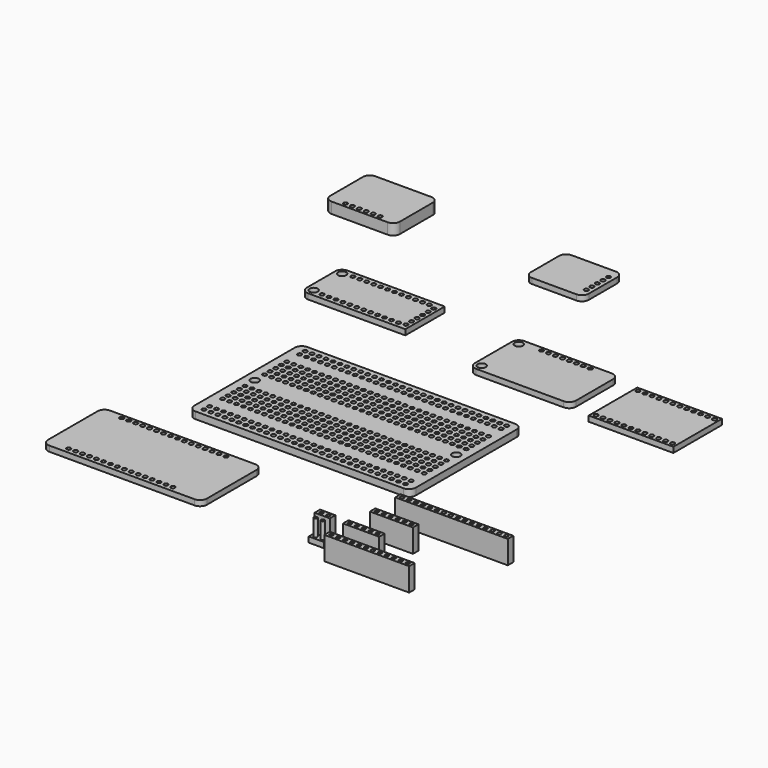
from build123d import *

# Parameters (mm, degrees)
F0_W      = 81
F0_H      = 51
F0_R      = 0.75
F0_R_2    = 1.5
F1_DEPTH  = 2.5
F2_R      = 2.5
F3_W      = 5.58
F3_H      = 2.5
F3_R      = 0.625
F4_DEPTH  = 8.5
F5_DEPTH  = 2
F6_W      = 37
F6_H      = 22
F6_R      = 1.5
F6_R_2    = 0.75
F7_DEPTH  = 2
F8_R      = 2.5
F3_W_2    = 13.2
F9_DEPTH  = 8.5
F6_W_2    = 38
F6_H_2    = 18
F10_DEPTH = 2
F11_R     = 2.5
F3_W_3    = 30.98
F12_DEPTH = 8.5
F6_W_3    = 58.08
F6_H_3    = 27.72
F13_DEPTH = 2
F14_R     = 2.54
F6_W_4    = 21.2070047855
F15_DEPTH = 2
F16_R     = 2.5
F6_W_5    = 25.5
F6_H_4    = 20
F17_DEPTH = 4
F18_R     = 2.5
F6_W_6    = 30.9399995804
F6_H_5    = 22.16
F19_DEPTH = 2
F3_W_4    = 15.74
F20_DEPTH = 8.5
F21_DEPTH = 8
F3_W_5    = 41.14
F3_R_2    = 0.6724855027
F22_DEPTH = 8.5


# Not quite as in the source:
# - a feature names something its author has since deleted; it is built from what else it names


with BuildPart() as f1:
    # F0 (on Top) → F1 (new body)
    with BuildSketch(Plane.XY):
        with Locations((2.4331173706, -0.0898422903)):
            Rectangle(F0_W, F0_H)
        with Locations((-34.3968826294, -23.1898422903)):
            Circle(F0_R, mode=Mode.SUBTRACT)
        with Locations((-31.8568826675, -23.1898422903)):
            Circle(F0_R, mode=Mode.SUBTRACT)
        with Locations((-29.3168827057, -23.1898422903)):
            Circle(F0_R, mode=Mode.SUBTRACT)
        with Locations((-34.3968826772, -20.6498423284)):
            Circle(F0_R, mode=Mode.SUBTRACT)
        with Locations((-31.8568827154, -20.6498423284)):
            Circle(F0_R, mode=Mode.SUBTRACT)
        with Locations((-29.3168827535, -20.6498423284)):
            Circle(F0_R, mode=Mode.SUBTRACT)
        with Locations((-26.7768827438, -23.1898422903)):
            Circle(F0_R, mode=Mode.SUBTRACT)
        with Locations((-24.236882782, -23.1898422903)):
            Circle(F0_R, mode=Mode.SUBTRACT)
        with Locations((-21.6968828201, -23.1898422903)):
            Circle(F0_R, mode=Mode.SUBTRACT)
        with Locations((-19.1568828583, -23.1898422903)):
            Circle(F0_R, mode=Mode.SUBTRACT)
        with Locations((-26.7768827917, -20.6498423284)):
            Circle(F0_R, mode=Mode.SUBTRACT)
        with Locations((-24.2368828298, -20.6498423284)):
            Circle(F0_R, mode=Mode.SUBTRACT)
        with Locations((-21.696882868, -20.6498423284)):
            Circle(F0_R, mode=Mode.SUBTRACT)
        with Locations((-19.1568829061, -20.6498423284)):
            Circle(F0_R, mode=Mode.SUBTRACT)
        with Locations((-34.3968826584, -14.6599998474)):
            Circle(F0_R, mode=Mode.SUBTRACT)
        with Locations((-31.8568826966, -14.6599998474)):
            Circle(F0_R, mode=Mode.SUBTRACT)
        with Locations((-29.3168827347, -14.6599998474)):
            Circle(F0_R, mode=Mode.SUBTRACT)
        with Locations((-26.7768827729, -14.6599998474)):
            Circle(F0_R, mode=Mode.SUBTRACT)
        with Locations((-24.236882811, -14.6599998474)):
            Circle(F0_R, mode=Mode.SUBTRACT)
        with Locations((-21.6968828492, -14.6599998474)):
            Circle(F0_R, mode=Mode.SUBTRACT)
        with Locations((-19.1568828873, -14.6599998474)):
            Circle(F0_R, mode=Mode.SUBTRACT)
        with Locations((-16.6168828964, -23.1898422903)):
            Circle(F0_R, mode=Mode.SUBTRACT)
        with Locations((-14.0768829346, -23.1898422903)):
            Circle(F0_R, mode=Mode.SUBTRACT)
        with Locations((-11.5368829727, -23.1898422903)):
            Circle(F0_R, mode=Mode.SUBTRACT)
        with Locations((-8.9968830109, -23.1898422903)):
            Circle(F0_R, mode=Mode.SUBTRACT)
        with Locations((-16.6168829443, -20.6498423284)):
            Circle(F0_R, mode=Mode.SUBTRACT)
        with Locations((-14.0768829824, -20.6498423284)):
            Circle(F0_R, mode=Mode.SUBTRACT)
        with Locations((-11.5368830206, -20.6498423284)):
            Circle(F0_R, mode=Mode.SUBTRACT)
        with Locations((-8.9968830587, -20.6498423284)):
            Circle(F0_R, mode=Mode.SUBTRACT)
        with Locations((-6.456883049, -23.1898422903)):
            Circle(F0_R, mode=Mode.SUBTRACT)
        with Locations((-3.9168830872, -23.1898422903)):
            Circle(F0_R, mode=Mode.SUBTRACT)
        with Locations((-1.3768831253, -23.1898422903)):
            Circle(F0_R, mode=Mode.SUBTRACT)
        with Locations((1.1631168365, -23.1898422903)):
            Circle(F0_R, mode=Mode.SUBTRACT)
        with Locations((-6.4568830969, -20.6498423284)):
            Circle(F0_R, mode=Mode.SUBTRACT)
        with Locations((-3.916883135, -20.6498423284)):
            Circle(F0_R, mode=Mode.SUBTRACT)
        with Locations((-1.3768831731, -20.6498423284)):
            Circle(F0_R, mode=Mode.SUBTRACT)
        with Locations((1.1631167887, -20.6498423284)):
            Circle(F0_R, mode=Mode.SUBTRACT)
        with Locations((-16.6168829255, -14.6599998474)):
            Circle(F0_R, mode=Mode.SUBTRACT)
        with Locations((-14.0768829636, -14.6599998474)):
            Circle(F0_R, mode=Mode.SUBTRACT)
        with Locations((-11.5368830018, -14.6599998474)):
            Circle(F0_R, mode=Mode.SUBTRACT)
        with Locations((-8.9968830399, -14.6599998474)):
            Circle(F0_R, mode=Mode.SUBTRACT)
        with Locations((-6.4568830781, -14.6599998474)):
            Circle(F0_R, mode=Mode.SUBTRACT)
        with Locations((-3.9168831162, -14.6599998474)):
            Circle(F0_R, mode=Mode.SUBTRACT)
        with Locations((-1.3768831544, -14.6599998474)):
            Circle(F0_R, mode=Mode.SUBTRACT)
        with Locations((1.1631168075, -14.6599998474)):
            Circle(F0_R, mode=Mode.SUBTRACT)
        with Locations((-34.3968826584, -12.1199998856)):
            Circle(F0_R, mode=Mode.SUBTRACT)
        with Locations((-31.8568826966, -12.1199998856)):
            Circle(F0_R, mode=Mode.SUBTRACT)
        with Locations((-29.3168827347, -12.1199998856)):
            Circle(F0_R, mode=Mode.SUBTRACT)
        with Locations((-34.3968826584, -9.5799999237)):
            Circle(F0_R, mode=Mode.SUBTRACT)
        with Locations((-34.3968826584, -7.0399999619)):
            Circle(F0_R, mode=Mode.SUBTRACT)
        with Locations((-31.8568826966, -9.5799999237)):
            Circle(F0_R, mode=Mode.SUBTRACT)
        with Locations((-29.3168827347, -9.5799999237)):
            Circle(F0_R, mode=Mode.SUBTRACT)
        with Locations((-31.8568826966, -7.0399999619)):
            Circle(F0_R, mode=Mode.SUBTRACT)
        with Locations((-29.3168827347, -7.0399999619)):
            Circle(F0_R, mode=Mode.SUBTRACT)
        with Locations((-26.7768827729, -12.1199998856)):
            Circle(F0_R, mode=Mode.SUBTRACT)
        with Locations((-24.236882811, -12.1199998856)):
            Circle(F0_R, mode=Mode.SUBTRACT)
        with Locations((-21.6968828492, -12.1199998856)):
            Circle(F0_R, mode=Mode.SUBTRACT)
        with Locations((-19.1568828873, -12.1199998856)):
            Circle(F0_R, mode=Mode.SUBTRACT)
        with Locations((-26.7768827729, -9.5799999237)):
            Circle(F0_R, mode=Mode.SUBTRACT)
        with Locations((-24.236882811, -9.5799999237)):
            Circle(F0_R, mode=Mode.SUBTRACT)
        with Locations((-26.7768827729, -7.0399999619)):
            Circle(F0_R, mode=Mode.SUBTRACT)
        with Locations((-24.236882811, -7.0399999619)):
            Circle(F0_R, mode=Mode.SUBTRACT)
        with Locations((-21.6968828492, -9.5799999237)):
            Circle(F0_R, mode=Mode.SUBTRACT)
        with Locations((-19.1568828873, -9.5799999237)):
            Circle(F0_R, mode=Mode.SUBTRACT)
        with Locations((-21.6968828492, -7.0399999619)):
            Circle(F0_R, mode=Mode.SUBTRACT)
        with Locations((-19.1568828873, -7.0399999619)):
            Circle(F0_R, mode=Mode.SUBTRACT)
        with Locations((-34.3968826584, -4.5)):
            Circle(F0_R, mode=Mode.SUBTRACT)
        with Locations((-31.8568826966, -4.5)):
            Circle(F0_R, mode=Mode.SUBTRACT)
        with Locations((-29.3168827347, -4.5)):
            Circle(F0_R, mode=Mode.SUBTRACT)
        with Locations((-26.7768827729, -4.5)):
            Circle(F0_R, mode=Mode.SUBTRACT)
        with Locations((-24.236882811, -4.5)):
            Circle(F0_R, mode=Mode.SUBTRACT)
        with Locations((-21.6968828492, -4.5)):
            Circle(F0_R, mode=Mode.SUBTRACT)
        with Locations((-19.1568828873, -4.5)):
            Circle(F0_R, mode=Mode.SUBTRACT)
        with Locations((-16.6168829255, -12.1199998856)):
            Circle(F0_R, mode=Mode.SUBTRACT)
        with Locations((-14.0768829636, -12.1199998856)):
            Circle(F0_R, mode=Mode.SUBTRACT)
        with Locations((-11.5368830018, -12.1199998856)):
            Circle(F0_R, mode=Mode.SUBTRACT)
        with Locations((-8.9968830399, -12.1199998856)):
            Circle(F0_R, mode=Mode.SUBTRACT)
        with Locations((-16.6168829255, -9.5799999237)):
            Circle(F0_R, mode=Mode.SUBTRACT)
        with Locations((-14.0768829636, -9.5799999237)):
            Circle(F0_R, mode=Mode.SUBTRACT)
        with Locations((-16.6168829255, -7.0399999619)):
            Circle(F0_R, mode=Mode.SUBTRACT)
        with Locations((-14.0768829636, -7.0399999619)):
            Circle(F0_R, mode=Mode.SUBTRACT)
        with Locations((-11.5368830018, -9.5799999237)):
            Circle(F0_R, mode=Mode.SUBTRACT)
        with Locations((-8.9968830399, -9.5799999237)):
            Circle(F0_R, mode=Mode.SUBTRACT)
        with Locations((-11.5368830018, -7.0399999619)):
            Circle(F0_R, mode=Mode.SUBTRACT)
        with Locations((-8.9968830399, -7.0399999619)):
            Circle(F0_R, mode=Mode.SUBTRACT)
        with Locations((-6.4568830781, -12.1199998856)):
            Circle(F0_R, mode=Mode.SUBTRACT)
        with Locations((-3.9168831162, -12.1199998856)):
            Circle(F0_R, mode=Mode.SUBTRACT)
        with Locations((-1.3768831544, -12.1199998856)):
            Circle(F0_R, mode=Mode.SUBTRACT)
        with Locations((1.1631168075, -12.1199998856)):
            Circle(F0_R, mode=Mode.SUBTRACT)
        with Locations((-6.4568830781, -9.5799999237)):
            Circle(F0_R, mode=Mode.SUBTRACT)
        with Locations((-3.9168831162, -9.5799999237)):
            Circle(F0_R, mode=Mode.SUBTRACT)
        with Locations((-6.4568830781, -7.0399999619)):
            Circle(F0_R, mode=Mode.SUBTRACT)
        with Locations((-3.9168831162, -7.0399999619)):
            Circle(F0_R, mode=Mode.SUBTRACT)
        with Locations((-1.3768831544, -9.5799999237)):
            Circle(F0_R, mode=Mode.SUBTRACT)
        with Locations((1.1631168075, -9.5799999237)):
            Circle(F0_R, mode=Mode.SUBTRACT)
        with Locations((-1.3768831544, -7.0399999619)):
            Circle(F0_R, mode=Mode.SUBTRACT)
        with Locations((1.1631168075, -7.0399999619)):
            Circle(F0_R, mode=Mode.SUBTRACT)
        with Locations((-16.6168829255, -4.5)):
            Circle(F0_R, mode=Mode.SUBTRACT)
        with Locations((-14.0768829636, -4.5)):
            Circle(F0_R, mode=Mode.SUBTRACT)
        with Locations((-11.5368830018, -4.5)):
            Circle(F0_R, mode=Mode.SUBTRACT)
        with Locations((-8.9968830399, -4.5)):
            Circle(F0_R, mode=Mode.SUBTRACT)
        with Locations((-6.4568830781, -4.5)):
            Circle(F0_R, mode=Mode.SUBTRACT)
        with Locations((-3.9168831162, -4.5)):
            Circle(F0_R, mode=Mode.SUBTRACT)
        with Locations((-1.3768831544, -4.5)):
            Circle(F0_R, mode=Mode.SUBTRACT)
        with Locations((1.1631168075, -4.5)):
            Circle(F0_R, mode=Mode.SUBTRACT)
        with Locations((3.7031167984, -23.1898422903)):
            Circle(F0_R, mode=Mode.SUBTRACT)
        with Locations((6.2431167603, -23.1898422903)):
            Circle(F0_R, mode=Mode.SUBTRACT)
        with Locations((8.7831167221, -23.1898422903)):
            Circle(F0_R, mode=Mode.SUBTRACT)
        with Locations((11.323116684, -23.1898422903)):
            Circle(F0_R, mode=Mode.SUBTRACT)
        with Locations((3.7031167506, -20.6498423284)):
            Circle(F0_R, mode=Mode.SUBTRACT)
        with Locations((6.2431167124, -20.6498423284)):
            Circle(F0_R, mode=Mode.SUBTRACT)
        with Locations((8.7831166743, -20.6498423284)):
            Circle(F0_R, mode=Mode.SUBTRACT)
        with Locations((11.3231166361, -20.6498423284)):
            Circle(F0_R, mode=Mode.SUBTRACT)
        with Locations((13.8631166458, -23.1898422903)):
            Circle(F0_R, mode=Mode.SUBTRACT)
        with Locations((16.4031166077, -23.1898422903)):
            Circle(F0_R, mode=Mode.SUBTRACT)
        with Locations((18.9431165695, -23.1898422903)):
            Circle(F0_R, mode=Mode.SUBTRACT)
        with Locations((21.4831165314, -23.1898422903)):
            Circle(F0_R, mode=Mode.SUBTRACT)
        with Locations((13.863116598, -20.6498423284)):
            Circle(F0_R, mode=Mode.SUBTRACT)
        with Locations((16.4031165598, -20.6498423284)):
            Circle(F0_R, mode=Mode.SUBTRACT)
        with Locations((18.9431165217, -20.6498423284)):
            Circle(F0_R, mode=Mode.SUBTRACT)
        with Locations((21.4831164835, -20.6498423284)):
            Circle(F0_R, mode=Mode.SUBTRACT)
        with Locations((3.7031167693, -14.6599998474)):
            Circle(F0_R, mode=Mode.SUBTRACT)
        with Locations((6.2431167312, -14.6599998474)):
            Circle(F0_R, mode=Mode.SUBTRACT)
        with Locations((8.7831166931, -14.6599998474)):
            Circle(F0_R, mode=Mode.SUBTRACT)
        with Locations((11.3231166549, -14.6599998474)):
            Circle(F0_R, mode=Mode.SUBTRACT)
        with Locations((13.8631166168, -14.6599998474)):
            Circle(F0_R, mode=Mode.SUBTRACT)
        with Locations((16.4031165786, -14.6599998474)):
            Circle(F0_R, mode=Mode.SUBTRACT)
        with Locations((18.9431165405, -14.6599998474)):
            Circle(F0_R, mode=Mode.SUBTRACT)
        with Locations((21.4831165023, -14.6599998474)):
            Circle(F0_R, mode=Mode.SUBTRACT)
        with Locations((24.0231164932, -23.1898422903)):
            Circle(F0_R, mode=Mode.SUBTRACT)
        with Locations((26.5631164551, -23.1898422903)):
            Circle(F0_R, mode=Mode.SUBTRACT)
        with Locations((29.1031164169, -23.1898422903)):
            Circle(F0_R, mode=Mode.SUBTRACT)
        with Locations((31.6431163788, -23.1898422903)):
            Circle(F0_R, mode=Mode.SUBTRACT)
        with Locations((24.0231164454, -20.6498423284)):
            Circle(F0_R, mode=Mode.SUBTRACT)
        with Locations((26.5631164072, -20.6498423284)):
            Circle(F0_R, mode=Mode.SUBTRACT)
        with Locations((29.1031163691, -20.6498423284)):
            Circle(F0_R, mode=Mode.SUBTRACT)
        with Locations((31.6431163309, -20.6498423284)):
            Circle(F0_R, mode=Mode.SUBTRACT)
        with Locations((34.1831163406, -23.1898422903)):
            Circle(F0_R, mode=Mode.SUBTRACT)
        with Locations((36.7231163025, -23.1898422903)):
            Circle(F0_R, mode=Mode.SUBTRACT)
        with Locations((39.2631162643, -23.1898422903)):
            Circle(F0_R, mode=Mode.SUBTRACT)
        with Locations((34.1831162928, -20.6498423284)):
            Circle(F0_R, mode=Mode.SUBTRACT)
        with Locations((36.7231162546, -20.6498423284)):
            Circle(F0_R, mode=Mode.SUBTRACT)
        with Locations((39.2631162165, -20.6498423284)):
            Circle(F0_R, mode=Mode.SUBTRACT)
        with Locations((24.0231164642, -14.6599998474)):
            Circle(F0_R, mode=Mode.SUBTRACT)
        with Locations((26.563116426, -14.6599998474)):
            Circle(F0_R, mode=Mode.SUBTRACT)
        with Locations((29.1031163879, -14.6599998474)):
            Circle(F0_R, mode=Mode.SUBTRACT)
        with Locations((31.6431163497, -14.6599998474)):
            Circle(F0_R, mode=Mode.SUBTRACT)
        with Locations((34.1831163116, -14.6599998474)):
            Circle(F0_R, mode=Mode.SUBTRACT)
        with Locations((36.7231162734, -14.6599998474)):
            Circle(F0_R, mode=Mode.SUBTRACT)
        with Locations((39.2631162353, -14.6599998474)):
            Circle(F0_R, mode=Mode.SUBTRACT)
        with Locations((3.7031167693, -12.1199998856)):
            Circle(F0_R, mode=Mode.SUBTRACT)
        with Locations((6.2431167312, -12.1199998856)):
            Circle(F0_R, mode=Mode.SUBTRACT)
        with Locations((8.7831166931, -12.1199998856)):
            Circle(F0_R, mode=Mode.SUBTRACT)
        with Locations((11.3231166549, -12.1199998856)):
            Circle(F0_R, mode=Mode.SUBTRACT)
        with Locations((3.7031167693, -9.5799999237)):
            Circle(F0_R, mode=Mode.SUBTRACT)
        with Locations((6.2431167312, -9.5799999237)):
            Circle(F0_R, mode=Mode.SUBTRACT)
        with Locations((3.7031167693, -7.0399999619)):
            Circle(F0_R, mode=Mode.SUBTRACT)
        with Locations((6.2431167312, -7.0399999619)):
            Circle(F0_R, mode=Mode.SUBTRACT)
        with Locations((8.7831166931, -9.5799999237)):
            Circle(F0_R, mode=Mode.SUBTRACT)
        with Locations((11.3231166549, -9.5799999237)):
            Circle(F0_R, mode=Mode.SUBTRACT)
        with Locations((8.7831166931, -7.0399999619)):
            Circle(F0_R, mode=Mode.SUBTRACT)
        with Locations((11.3231166549, -7.0399999619)):
            Circle(F0_R, mode=Mode.SUBTRACT)
        with Locations((13.8631166168, -12.1199998856)):
            Circle(F0_R, mode=Mode.SUBTRACT)
        with Locations((16.4031165786, -12.1199998856)):
            Circle(F0_R, mode=Mode.SUBTRACT)
        with Locations((18.9431165405, -12.1199998856)):
            Circle(F0_R, mode=Mode.SUBTRACT)
        with Locations((21.4831165023, -12.1199998856)):
            Circle(F0_R, mode=Mode.SUBTRACT)
        with Locations((13.8631166168, -9.5799999237)):
            Circle(F0_R, mode=Mode.SUBTRACT)
        with Locations((16.4031165786, -9.5799999237)):
            Circle(F0_R, mode=Mode.SUBTRACT)
        with Locations((13.8631166168, -7.0399999619)):
            Circle(F0_R, mode=Mode.SUBTRACT)
        with Locations((16.4031165786, -7.0399999619)):
            Circle(F0_R, mode=Mode.SUBTRACT)
        with Locations((18.9431165405, -9.5799999237)):
            Circle(F0_R, mode=Mode.SUBTRACT)
        with Locations((21.4831165023, -9.5799999237)):
            Circle(F0_R, mode=Mode.SUBTRACT)
        with Locations((18.9431165405, -7.0399999619)):
            Circle(F0_R, mode=Mode.SUBTRACT)
        with Locations((21.4831165023, -7.0399999619)):
            Circle(F0_R, mode=Mode.SUBTRACT)
        with Locations((3.7031167693, -4.5)):
            Circle(F0_R, mode=Mode.SUBTRACT)
        with Locations((6.2431167312, -4.5)):
            Circle(F0_R, mode=Mode.SUBTRACT)
        with Locations((8.7831166931, -4.5)):
            Circle(F0_R, mode=Mode.SUBTRACT)
        with Locations((11.3231166549, -4.5)):
            Circle(F0_R, mode=Mode.SUBTRACT)
        with Locations((13.8631166168, -4.5)):
            Circle(F0_R, mode=Mode.SUBTRACT)
        with Locations((16.4031165786, -4.5)):
            Circle(F0_R, mode=Mode.SUBTRACT)
        with Locations((18.9431165405, -4.5)):
            Circle(F0_R, mode=Mode.SUBTRACT)
        with Locations((21.4831165023, -4.5)):
            Circle(F0_R, mode=Mode.SUBTRACT)
        with Locations((24.0231164642, -12.1199998856)):
            Circle(F0_R, mode=Mode.SUBTRACT)
        with Locations((26.563116426, -12.1199998856)):
            Circle(F0_R, mode=Mode.SUBTRACT)
        with Locations((29.1031163879, -12.1199998856)):
            Circle(F0_R, mode=Mode.SUBTRACT)
        with Locations((31.6431163497, -12.1199998856)):
            Circle(F0_R, mode=Mode.SUBTRACT)
        with Locations((24.0231164642, -9.5799999237)):
            Circle(F0_R, mode=Mode.SUBTRACT)
        with Locations((26.563116426, -9.5799999237)):
            Circle(F0_R, mode=Mode.SUBTRACT)
        with Locations((24.0231164642, -7.0399999619)):
            Circle(F0_R, mode=Mode.SUBTRACT)
        with Locations((26.563116426, -7.0399999619)):
            Circle(F0_R, mode=Mode.SUBTRACT)
        with Locations((29.1031163879, -9.5799999237)):
            Circle(F0_R, mode=Mode.SUBTRACT)
        with Locations((31.6431163497, -9.5799999237)):
            Circle(F0_R, mode=Mode.SUBTRACT)
        with Locations((29.1031163879, -7.0399999619)):
            Circle(F0_R, mode=Mode.SUBTRACT)
        with Locations((31.6431163497, -7.0399999619)):
            Circle(F0_R, mode=Mode.SUBTRACT)
        with Locations((34.1831163116, -12.1199998856)):
            Circle(F0_R, mode=Mode.SUBTRACT)
        with Locations((36.7231162734, -12.1199998856)):
            Circle(F0_R, mode=Mode.SUBTRACT)
        with Locations((39.2631162353, -12.1199998856)):
            Circle(F0_R, mode=Mode.SUBTRACT)
        with Locations((34.1831163116, -9.5799999237)):
            Circle(F0_R, mode=Mode.SUBTRACT)
        with Locations((36.7231162734, -9.5799999237)):
            Circle(F0_R, mode=Mode.SUBTRACT)
        with Locations((34.1831163116, -7.0399999619)):
            Circle(F0_R, mode=Mode.SUBTRACT)
        with Locations((36.7231162734, -7.0399999619)):
            Circle(F0_R, mode=Mode.SUBTRACT)
        with Locations((39.2631162353, -9.5799999237)):
            Circle(F0_R, mode=Mode.SUBTRACT)
        with Locations((39.2631162353, -7.0399999619)):
            Circle(F0_R, mode=Mode.SUBTRACT)
        with Locations((24.0231164642, -4.5)):
            Circle(F0_R, mode=Mode.SUBTRACT)
        with Locations((26.563116426, -4.5)):
            Circle(F0_R, mode=Mode.SUBTRACT)
        with Locations((29.1031163879, -4.5)):
            Circle(F0_R, mode=Mode.SUBTRACT)
        with Locations((31.6431163497, -4.5)):
            Circle(F0_R, mode=Mode.SUBTRACT)
        with Locations((34.1831163116, -4.5)):
            Circle(F0_R, mode=Mode.SUBTRACT)
        with Locations((36.7231162734, -4.5)):
            Circle(F0_R, mode=Mode.SUBTRACT)
        with Locations((39.2631162353, -4.5)):
            Circle(F0_R, mode=Mode.SUBTRACT)
        with Locations((-34.3968826532, 0)):
            Circle(F0_R_2, mode=Mode.SUBTRACT)
        with Locations((-34.396882648, 4.5)):
            Circle(F0_R, mode=Mode.SUBTRACT)
        with Locations((-31.8568826861, 4.5)):
            Circle(F0_R, mode=Mode.SUBTRACT)
        with Locations((-29.3168827243, 4.5)):
            Circle(F0_R, mode=Mode.SUBTRACT)
        with Locations((-26.7768827624, 4.5)):
            Circle(F0_R, mode=Mode.SUBTRACT)
        with Locations((-24.2368828006, 4.5)):
            Circle(F0_R, mode=Mode.SUBTRACT)
        with Locations((-21.6968828387, 4.5)):
            Circle(F0_R, mode=Mode.SUBTRACT)
        with Locations((-19.1568828769, 4.5)):
            Circle(F0_R, mode=Mode.SUBTRACT)
        with Locations((-34.396882648, 7.0399999619)):
            Circle(F0_R, mode=Mode.SUBTRACT)
        with Locations((-31.8568826861, 7.0399999619)):
            Circle(F0_R, mode=Mode.SUBTRACT)
        with Locations((-29.3168827243, 7.0399999619)):
            Circle(F0_R, mode=Mode.SUBTRACT)
        with Locations((-34.396882648, 9.5799999237)):
            Circle(F0_R, mode=Mode.SUBTRACT)
        with Locations((-34.396882648, 12.1199998856)):
            Circle(F0_R, mode=Mode.SUBTRACT)
        with Locations((-31.8568826861, 9.5799999237)):
            Circle(F0_R, mode=Mode.SUBTRACT)
        with Locations((-29.3168827243, 9.5799999237)):
            Circle(F0_R, mode=Mode.SUBTRACT)
        with Locations((-31.8568826861, 12.1199998856)):
            Circle(F0_R, mode=Mode.SUBTRACT)
        with Locations((-29.3168827243, 12.1199998856)):
            Circle(F0_R, mode=Mode.SUBTRACT)
        with Locations((-26.7768827624, 7.0399999619)):
            Circle(F0_R, mode=Mode.SUBTRACT)
        with Locations((-24.2368828006, 7.0399999619)):
            Circle(F0_R, mode=Mode.SUBTRACT)
        with Locations((-21.6968828387, 7.0399999619)):
            Circle(F0_R, mode=Mode.SUBTRACT)
        with Locations((-19.1568828769, 7.0399999619)):
            Circle(F0_R, mode=Mode.SUBTRACT)
        with Locations((-26.7768827624, 9.5799999237)):
            Circle(F0_R, mode=Mode.SUBTRACT)
        with Locations((-24.2368828006, 9.5799999237)):
            Circle(F0_R, mode=Mode.SUBTRACT)
        with Locations((-26.7768827624, 12.1199998856)):
            Circle(F0_R, mode=Mode.SUBTRACT)
        with Locations((-24.2368828006, 12.1199998856)):
            Circle(F0_R, mode=Mode.SUBTRACT)
        with Locations((-21.6968828387, 9.5799999237)):
            Circle(F0_R, mode=Mode.SUBTRACT)
        with Locations((-19.1568828769, 9.5799999237)):
            Circle(F0_R, mode=Mode.SUBTRACT)
        with Locations((-21.6968828387, 12.1199998856)):
            Circle(F0_R, mode=Mode.SUBTRACT)
        with Locations((-19.1568828769, 12.1199998856)):
            Circle(F0_R, mode=Mode.SUBTRACT)
        with Locations((-16.616882915, 4.5)):
            Circle(F0_R, mode=Mode.SUBTRACT)
        with Locations((-14.0768829532, 4.5)):
            Circle(F0_R, mode=Mode.SUBTRACT)
        with Locations((-11.5368829913, 4.5)):
            Circle(F0_R, mode=Mode.SUBTRACT)
        with Locations((-8.9968830294, 4.5)):
            Circle(F0_R, mode=Mode.SUBTRACT)
        with Locations((-6.4568830676, 4.5)):
            Circle(F0_R, mode=Mode.SUBTRACT)
        with Locations((-3.9168831057, 4.5)):
            Circle(F0_R, mode=Mode.SUBTRACT)
        with Locations((-1.3768831439, 4.5)):
            Circle(F0_R, mode=Mode.SUBTRACT)
        with Locations((1.163116818, 4.5)):
            Circle(F0_R, mode=Mode.SUBTRACT)
        with Locations((-16.616882915, 7.0399999619)):
            Circle(F0_R, mode=Mode.SUBTRACT)
        with Locations((-14.0768829532, 7.0399999619)):
            Circle(F0_R, mode=Mode.SUBTRACT)
        with Locations((-11.5368829913, 7.0399999619)):
            Circle(F0_R, mode=Mode.SUBTRACT)
        with Locations((-8.9968830294, 7.0399999619)):
            Circle(F0_R, mode=Mode.SUBTRACT)
        with Locations((-16.616882915, 9.5799999237)):
            Circle(F0_R, mode=Mode.SUBTRACT)
        with Locations((-14.0768829532, 9.5799999237)):
            Circle(F0_R, mode=Mode.SUBTRACT)
        with Locations((-16.616882915, 12.1199998856)):
            Circle(F0_R, mode=Mode.SUBTRACT)
        with Locations((-14.0768829532, 12.1199998856)):
            Circle(F0_R, mode=Mode.SUBTRACT)
        with Locations((-11.5368829913, 9.5799999237)):
            Circle(F0_R, mode=Mode.SUBTRACT)
        with Locations((-8.9968830294, 9.5799999237)):
            Circle(F0_R, mode=Mode.SUBTRACT)
        with Locations((-11.5368829913, 12.1199998856)):
            Circle(F0_R, mode=Mode.SUBTRACT)
        with Locations((-8.9968830294, 12.1199998856)):
            Circle(F0_R, mode=Mode.SUBTRACT)
        with Locations((-6.4568830676, 7.0399999619)):
            Circle(F0_R, mode=Mode.SUBTRACT)
        with Locations((-3.9168831057, 7.0399999619)):
            Circle(F0_R, mode=Mode.SUBTRACT)
        with Locations((-1.3768831439, 7.0399999619)):
            Circle(F0_R, mode=Mode.SUBTRACT)
        with Locations((1.163116818, 7.0399999619)):
            Circle(F0_R, mode=Mode.SUBTRACT)
        with Locations((-6.4568830676, 9.5799999237)):
            Circle(F0_R, mode=Mode.SUBTRACT)
        with Locations((-3.9168831057, 9.5799999237)):
            Circle(F0_R, mode=Mode.SUBTRACT)
        with Locations((-6.4568830676, 12.1199998856)):
            Circle(F0_R, mode=Mode.SUBTRACT)
        with Locations((-3.9168831057, 12.1199998856)):
            Circle(F0_R, mode=Mode.SUBTRACT)
        with Locations((-1.3768831439, 9.5799999237)):
            Circle(F0_R, mode=Mode.SUBTRACT)
        with Locations((1.163116818, 9.5799999237)):
            Circle(F0_R, mode=Mode.SUBTRACT)
        with Locations((-1.3768831439, 12.1199998856)):
            Circle(F0_R, mode=Mode.SUBTRACT)
        with Locations((1.163116818, 12.1199998856)):
            Circle(F0_R, mode=Mode.SUBTRACT)
        with Locations((-34.396882648, 14.6599998474)):
            Circle(F0_R, mode=Mode.SUBTRACT)
        with Locations((-31.8568826861, 14.6599998474)):
            Circle(F0_R, mode=Mode.SUBTRACT)
        with Locations((-29.3168827243, 14.6599998474)):
            Circle(F0_R, mode=Mode.SUBTRACT)
        with Locations((-26.7768827624, 14.6599998474)):
            Circle(F0_R, mode=Mode.SUBTRACT)
        with Locations((-24.2368828006, 14.6599998474)):
            Circle(F0_R, mode=Mode.SUBTRACT)
        with Locations((-21.6968828387, 14.6599998474)):
            Circle(F0_R, mode=Mode.SUBTRACT)
        with Locations((-19.1568828769, 14.6599998474)):
            Circle(F0_R, mode=Mode.SUBTRACT)
        with Locations((-34.3968826294, 20.4701577478)):
            Circle(F0_R, mode=Mode.SUBTRACT)
        with Locations((-31.8568826675, 20.4701577478)):
            Circle(F0_R, mode=Mode.SUBTRACT)
        with Locations((-29.3168827057, 20.4701577478)):
            Circle(F0_R, mode=Mode.SUBTRACT)
        with Locations((-34.3968826294, 23.0101577097)):
            Circle(F0_R, mode=Mode.SUBTRACT)
        with Locations((-31.8568826675, 23.0101577097)):
            Circle(F0_R, mode=Mode.SUBTRACT)
        with Locations((-29.3168827057, 23.0101577097)):
            Circle(F0_R, mode=Mode.SUBTRACT)
        with Locations((-26.7768827438, 20.4701577478)):
            Circle(F0_R, mode=Mode.SUBTRACT)
        with Locations((-24.236882782, 20.4701577478)):
            Circle(F0_R, mode=Mode.SUBTRACT)
        with Locations((-21.6968828201, 20.4701577478)):
            Circle(F0_R, mode=Mode.SUBTRACT)
        with Locations((-19.1568828583, 20.4701577478)):
            Circle(F0_R, mode=Mode.SUBTRACT)
        with Locations((-26.7768827438, 23.0101577097)):
            Circle(F0_R, mode=Mode.SUBTRACT)
        with Locations((-24.236882782, 23.0101577097)):
            Circle(F0_R, mode=Mode.SUBTRACT)
        with Locations((-21.6968828201, 23.0101577097)):
            Circle(F0_R, mode=Mode.SUBTRACT)
        with Locations((-19.1568828583, 23.0101577097)):
            Circle(F0_R, mode=Mode.SUBTRACT)
        with Locations((-16.616882915, 14.6599998474)):
            Circle(F0_R, mode=Mode.SUBTRACT)
        with Locations((-14.0768829532, 14.6599998474)):
            Circle(F0_R, mode=Mode.SUBTRACT)
        with Locations((-11.5368829913, 14.6599998474)):
            Circle(F0_R, mode=Mode.SUBTRACT)
        with Locations((-8.9968830294, 14.6599998474)):
            Circle(F0_R, mode=Mode.SUBTRACT)
        with Locations((-6.4568830676, 14.6599998474)):
            Circle(F0_R, mode=Mode.SUBTRACT)
        with Locations((-3.9168831057, 14.6599998474)):
            Circle(F0_R, mode=Mode.SUBTRACT)
        with Locations((-1.3768831439, 14.6599998474)):
            Circle(F0_R, mode=Mode.SUBTRACT)
        with Locations((1.163116818, 14.6599998474)):
            Circle(F0_R, mode=Mode.SUBTRACT)
        with Locations((-16.6168828964, 20.4701577478)):
            Circle(F0_R, mode=Mode.SUBTRACT)
        with Locations((-14.0768829346, 20.4701577478)):
            Circle(F0_R, mode=Mode.SUBTRACT)
        with Locations((-11.5368829727, 20.4701577478)):
            Circle(F0_R, mode=Mode.SUBTRACT)
        with Locations((-8.9968830109, 20.4701577478)):
            Circle(F0_R, mode=Mode.SUBTRACT)
        with Locations((-16.6168828964, 23.0101577097)):
            Circle(F0_R, mode=Mode.SUBTRACT)
        with Locations((-14.0768829346, 23.0101577097)):
            Circle(F0_R, mode=Mode.SUBTRACT)
        with Locations((-11.5368829727, 23.0101577097)):
            Circle(F0_R, mode=Mode.SUBTRACT)
        with Locations((-8.9968830109, 23.0101577097)):
            Circle(F0_R, mode=Mode.SUBTRACT)
        with Locations((-6.456883049, 20.4701577478)):
            Circle(F0_R, mode=Mode.SUBTRACT)
        with Locations((-3.9168830872, 20.4701577478)):
            Circle(F0_R, mode=Mode.SUBTRACT)
        with Locations((-1.3768831253, 20.4701577478)):
            Circle(F0_R, mode=Mode.SUBTRACT)
        with Locations((1.1631168365, 20.4701577478)):
            Circle(F0_R, mode=Mode.SUBTRACT)
        with Locations((-6.456883049, 23.0101577097)):
            Circle(F0_R, mode=Mode.SUBTRACT)
        with Locations((-3.9168830872, 23.0101577097)):
            Circle(F0_R, mode=Mode.SUBTRACT)
        with Locations((-1.3768831253, 23.0101577097)):
            Circle(F0_R, mode=Mode.SUBTRACT)
        with Locations((1.1631168365, 23.0101577097)):
            Circle(F0_R, mode=Mode.SUBTRACT)
        with Locations((3.7031167798, 4.5)):
            Circle(F0_R, mode=Mode.SUBTRACT)
        with Locations((6.2431167417, 4.5)):
            Circle(F0_R, mode=Mode.SUBTRACT)
        with Locations((8.7831167035, 4.5)):
            Circle(F0_R, mode=Mode.SUBTRACT)
        with Locations((11.3231166654, 4.5)):
            Circle(F0_R, mode=Mode.SUBTRACT)
        with Locations((13.8631166272, 4.5)):
            Circle(F0_R, mode=Mode.SUBTRACT)
        with Locations((16.4031165891, 4.5)):
            Circle(F0_R, mode=Mode.SUBTRACT)
        with Locations((18.9431165509, 4.5)):
            Circle(F0_R, mode=Mode.SUBTRACT)
        with Locations((21.4831165128, 4.5)):
            Circle(F0_R, mode=Mode.SUBTRACT)
        with Locations((3.7031167798, 7.0399999619)):
            Circle(F0_R, mode=Mode.SUBTRACT)
        with Locations((6.2431167417, 7.0399999619)):
            Circle(F0_R, mode=Mode.SUBTRACT)
        with Locations((8.7831167035, 7.0399999619)):
            Circle(F0_R, mode=Mode.SUBTRACT)
        with Locations((11.3231166654, 7.0399999619)):
            Circle(F0_R, mode=Mode.SUBTRACT)
        with Locations((3.7031167798, 9.5799999237)):
            Circle(F0_R, mode=Mode.SUBTRACT)
        with Locations((6.2431167417, 9.5799999237)):
            Circle(F0_R, mode=Mode.SUBTRACT)
        with Locations((3.7031167798, 12.1199998856)):
            Circle(F0_R, mode=Mode.SUBTRACT)
        with Locations((6.2431167417, 12.1199998856)):
            Circle(F0_R, mode=Mode.SUBTRACT)
        with Locations((8.7831167035, 9.5799999237)):
            Circle(F0_R, mode=Mode.SUBTRACT)
        with Locations((11.3231166654, 9.5799999237)):
            Circle(F0_R, mode=Mode.SUBTRACT)
        with Locations((8.7831167035, 12.1199998856)):
            Circle(F0_R, mode=Mode.SUBTRACT)
        with Locations((11.3231166654, 12.1199998856)):
            Circle(F0_R, mode=Mode.SUBTRACT)
        with Locations((13.8631166272, 7.0399999619)):
            Circle(F0_R, mode=Mode.SUBTRACT)
        with Locations((16.4031165891, 7.0399999619)):
            Circle(F0_R, mode=Mode.SUBTRACT)
        with Locations((18.9431165509, 7.0399999619)):
            Circle(F0_R, mode=Mode.SUBTRACT)
        with Locations((21.4831165128, 7.0399999619)):
            Circle(F0_R, mode=Mode.SUBTRACT)
        with Locations((13.8631166272, 9.5799999237)):
            Circle(F0_R, mode=Mode.SUBTRACT)
        with Locations((16.4031165891, 9.5799999237)):
            Circle(F0_R, mode=Mode.SUBTRACT)
        with Locations((13.8631166272, 12.1199998856)):
            Circle(F0_R, mode=Mode.SUBTRACT)
        with Locations((16.4031165891, 12.1199998856)):
            Circle(F0_R, mode=Mode.SUBTRACT)
        with Locations((18.9431165509, 9.5799999237)):
            Circle(F0_R, mode=Mode.SUBTRACT)
        with Locations((21.4831165128, 9.5799999237)):
            Circle(F0_R, mode=Mode.SUBTRACT)
        with Locations((18.9431165509, 12.1199998856)):
            Circle(F0_R, mode=Mode.SUBTRACT)
        with Locations((21.4831165128, 12.1199998856)):
            Circle(F0_R, mode=Mode.SUBTRACT)
        with Locations((24.0231164746, 4.5)):
            Circle(F0_R, mode=Mode.SUBTRACT)
        with Locations((26.5631164365, 4.5)):
            Circle(F0_R, mode=Mode.SUBTRACT)
        with Locations((29.1031163984, 4.5)):
            Circle(F0_R, mode=Mode.SUBTRACT)
        with Locations((31.6431163602, 4.5)):
            Circle(F0_R, mode=Mode.SUBTRACT)
        with Locations((39.2631162405, 0)):
            Circle(F0_R_2, mode=Mode.SUBTRACT)
        with Locations((34.1831163221, 4.5)):
            Circle(F0_R, mode=Mode.SUBTRACT)
        with Locations((36.7231162839, 4.5)):
            Circle(F0_R, mode=Mode.SUBTRACT)
        with Locations((39.2631162458, 4.5)):
            Circle(F0_R, mode=Mode.SUBTRACT)
        with Locations((24.0231164746, 7.0399999619)):
            Circle(F0_R, mode=Mode.SUBTRACT)
        with Locations((26.5631164365, 7.0399999619)):
            Circle(F0_R, mode=Mode.SUBTRACT)
        with Locations((29.1031163984, 7.0399999619)):
            Circle(F0_R, mode=Mode.SUBTRACT)
        with Locations((31.6431163602, 7.0399999619)):
            Circle(F0_R, mode=Mode.SUBTRACT)
        with Locations((24.0231164746, 9.5799999237)):
            Circle(F0_R, mode=Mode.SUBTRACT)
        with Locations((26.5631164365, 9.5799999237)):
            Circle(F0_R, mode=Mode.SUBTRACT)
        with Locations((24.0231164746, 12.1199998856)):
            Circle(F0_R, mode=Mode.SUBTRACT)
        with Locations((26.5631164365, 12.1199998856)):
            Circle(F0_R, mode=Mode.SUBTRACT)
        with Locations((29.1031163984, 9.5799999237)):
            Circle(F0_R, mode=Mode.SUBTRACT)
        with Locations((31.6431163602, 9.5799999237)):
            Circle(F0_R, mode=Mode.SUBTRACT)
        with Locations((29.1031163984, 12.1199998856)):
            Circle(F0_R, mode=Mode.SUBTRACT)
        with Locations((31.6431163602, 12.1199998856)):
            Circle(F0_R, mode=Mode.SUBTRACT)
        with Locations((34.1831163221, 7.0399999619)):
            Circle(F0_R, mode=Mode.SUBTRACT)
        with Locations((36.7231162839, 7.0399999619)):
            Circle(F0_R, mode=Mode.SUBTRACT)
        with Locations((39.2631162458, 7.0399999619)):
            Circle(F0_R, mode=Mode.SUBTRACT)
        with Locations((34.1831163221, 9.5799999237)):
            Circle(F0_R, mode=Mode.SUBTRACT)
        with Locations((36.7231162839, 9.5799999237)):
            Circle(F0_R, mode=Mode.SUBTRACT)
        with Locations((34.1831163221, 12.1199998856)):
            Circle(F0_R, mode=Mode.SUBTRACT)
        with Locations((36.7231162839, 12.1199998856)):
            Circle(F0_R, mode=Mode.SUBTRACT)
        with Locations((39.2631162458, 9.5799999237)):
            Circle(F0_R, mode=Mode.SUBTRACT)
        with Locations((39.2631162458, 12.1199998856)):
            Circle(F0_R, mode=Mode.SUBTRACT)
        with Locations((3.7031167798, 14.6599998474)):
            Circle(F0_R, mode=Mode.SUBTRACT)
        with Locations((6.2431167417, 14.6599998474)):
            Circle(F0_R, mode=Mode.SUBTRACT)
        with Locations((8.7831167035, 14.6599998474)):
            Circle(F0_R, mode=Mode.SUBTRACT)
        with Locations((11.3231166654, 14.6599998474)):
            Circle(F0_R, mode=Mode.SUBTRACT)
        with Locations((13.8631166272, 14.6599998474)):
            Circle(F0_R, mode=Mode.SUBTRACT)
        with Locations((16.4031165891, 14.6599998474)):
            Circle(F0_R, mode=Mode.SUBTRACT)
        with Locations((18.9431165509, 14.6599998474)):
            Circle(F0_R, mode=Mode.SUBTRACT)
        with Locations((21.4831165128, 14.6599998474)):
            Circle(F0_R, mode=Mode.SUBTRACT)
        with Locations((3.7031167984, 20.4701577478)):
            Circle(F0_R, mode=Mode.SUBTRACT)
        with Locations((6.2431167603, 20.4701577478)):
            Circle(F0_R, mode=Mode.SUBTRACT)
        with Locations((8.7831167221, 20.4701577478)):
            Circle(F0_R, mode=Mode.SUBTRACT)
        with Locations((11.323116684, 20.4701577478)):
            Circle(F0_R, mode=Mode.SUBTRACT)
        with Locations((3.7031167984, 23.0101577097)):
            Circle(F0_R, mode=Mode.SUBTRACT)
        with Locations((6.2431167603, 23.0101577097)):
            Circle(F0_R, mode=Mode.SUBTRACT)
        with Locations((8.7831167221, 23.0101577097)):
            Circle(F0_R, mode=Mode.SUBTRACT)
        with Locations((11.323116684, 23.0101577097)):
            Circle(F0_R, mode=Mode.SUBTRACT)
        with Locations((13.8631166458, 20.4701577478)):
            Circle(F0_R, mode=Mode.SUBTRACT)
        with Locations((16.4031166077, 20.4701577478)):
            Circle(F0_R, mode=Mode.SUBTRACT)
        with Locations((18.9431165695, 20.4701577478)):
            Circle(F0_R, mode=Mode.SUBTRACT)
        with Locations((21.4831165314, 20.4701577478)):
            Circle(F0_R, mode=Mode.SUBTRACT)
        with Locations((13.8631166458, 23.0101577097)):
            Circle(F0_R, mode=Mode.SUBTRACT)
        with Locations((16.4031166077, 23.0101577097)):
            Circle(F0_R, mode=Mode.SUBTRACT)
        with Locations((18.9431165695, 23.0101577097)):
            Circle(F0_R, mode=Mode.SUBTRACT)
        with Locations((21.4831165314, 23.0101577097)):
            Circle(F0_R, mode=Mode.SUBTRACT)
        with Locations((24.0231164746, 14.6599998474)):
            Circle(F0_R, mode=Mode.SUBTRACT)
        with Locations((26.5631164365, 14.6599998474)):
            Circle(F0_R, mode=Mode.SUBTRACT)
        with Locations((29.1031163984, 14.6599998474)):
            Circle(F0_R, mode=Mode.SUBTRACT)
        with Locations((31.6431163602, 14.6599998474)):
            Circle(F0_R, mode=Mode.SUBTRACT)
        with Locations((34.1831163221, 14.6599998474)):
            Circle(F0_R, mode=Mode.SUBTRACT)
        with Locations((36.7231162839, 14.6599998474)):
            Circle(F0_R, mode=Mode.SUBTRACT)
        with Locations((39.2631162458, 14.6599998474)):
            Circle(F0_R, mode=Mode.SUBTRACT)
        with Locations((24.0231164932, 20.4701577478)):
            Circle(F0_R, mode=Mode.SUBTRACT)
        with Locations((26.5631164551, 20.4701577478)):
            Circle(F0_R, mode=Mode.SUBTRACT)
        with Locations((29.1031164169, 20.4701577478)):
            Circle(F0_R, mode=Mode.SUBTRACT)
        with Locations((31.6431163788, 20.4701577478)):
            Circle(F0_R, mode=Mode.SUBTRACT)
        with Locations((24.0231164932, 23.0101577097)):
            Circle(F0_R, mode=Mode.SUBTRACT)
        with Locations((26.5631164551, 23.0101577097)):
            Circle(F0_R, mode=Mode.SUBTRACT)
        with Locations((29.1031164169, 23.0101577097)):
            Circle(F0_R, mode=Mode.SUBTRACT)
        with Locations((31.6431163788, 23.0101577097)):
            Circle(F0_R, mode=Mode.SUBTRACT)
        with Locations((34.1831163406, 20.4701577478)):
            Circle(F0_R, mode=Mode.SUBTRACT)
        with Locations((36.7231163025, 20.4701577478)):
            Circle(F0_R, mode=Mode.SUBTRACT)
        with Locations((39.2631162643, 20.4701577478)):
            Circle(F0_R, mode=Mode.SUBTRACT)
        with Locations((34.1831163406, 23.0101577097)):
            Circle(F0_R, mode=Mode.SUBTRACT)
        with Locations((36.7231163025, 23.0101577097)):
            Circle(F0_R, mode=Mode.SUBTRACT)
        with Locations((39.2631162643, 23.0101577097)):
            Circle(F0_R, mode=Mode.SUBTRACT)
    extrude(amount=F1_DEPTH)

    # F2
    f2_edges = [f1.edges().sort_by_distance(p)[0] for p in [
        (42.933117, 25.410158, 1.25),
        (42.933117, -25.589842, 1.25),
        (-38.066883, -25.589842, 1.25),
        (-38.066883, 25.410158, 1.25),
    ]]
    fillet(f2_edges, radius=F2_R)


with BuildPart() as f4:
    # F3 (on Top) → F4 (new body)
    with BuildSketch(Plane.XY):
        with Locations((40.0524000234, -60.9989538789)):
            Rectangle(F3_W, F3_H)
        with Locations((38.7824000234, -60.9989538789)):
            Circle(F3_R, mode=Mode.SUBTRACT)
        with Locations((41.3223999853, -60.9989538789)):
            Circle(F3_R, mode=Mode.SUBTRACT)
    extrude(amount=F4_DEPTH)


with BuildPart() as f5:
    # F3 (on Top) → F5 (new body)
    with BuildSketch(Plane.XY):
        with Locations((40.1041014385, -63.7300918698)):
            Rectangle(F3_W, F3_H)
        with Locations((38.8341014385, -63.7300918698)):
            Circle(F3_R, mode=Mode.SUBTRACT)
        with Locations((41.3741014004, -63.7300918698)):
            Circle(F3_R, mode=Mode.SUBTRACT)
    extrude(amount=F5_DEPTH)

    # F3 (on Top) → F21 (join)
    with BuildSketch(Plane.XY):
        with Locations((38.8341014385, -63.7300918698)):
            Circle(F3_R)
        with Locations((41.3741014004, -63.7300918698)):
            Circle(F3_R)
    extrude(amount=F21_DEPTH)


with BuildPart() as f7:
    # F6 (on Top) → F7 (new body)
    with BuildSketch(Plane.XY):
        with Locations((25.9184702337, 56.7231717071)):
            Rectangle(F6_W, F6_H)
        with Locations((9.9184702337, 48.2231717071)):
            Circle(F6_R, mode=Mode.SUBTRACT)
        with Locations((9.9184702337, 65.2231717071)):
            Circle(F6_R, mode=Mode.SUBTRACT)
        with Locations((17.4184702337, 66.2231717071)):
            Circle(F6_R_2, mode=Mode.SUBTRACT)
        with Locations((19.9584701955, 66.2231717071)):
            Circle(F6_R_2, mode=Mode.SUBTRACT)
        with Locations((22.4984701574, 66.2231717071)):
            Circle(F6_R_2, mode=Mode.SUBTRACT)
        with Locations((25.0384701192, 66.2231717071)):
            Circle(F6_R_2, mode=Mode.SUBTRACT)
        with Locations((27.5784700811, 66.2231717071)):
            Circle(F6_R_2, mode=Mode.SUBTRACT)
        with Locations((30.1184700429, 66.2231717071)):
            Circle(F6_R_2, mode=Mode.SUBTRACT)
        with Locations((32.6584700048, 66.2231717071)):
            Circle(F6_R_2, mode=Mode.SUBTRACT)
        with Locations((35.1984699667, 66.2231717071)):
            Circle(F6_R_2, mode=Mode.SUBTRACT)
    extrude(amount=F7_DEPTH)

    # F8
    f8_edges = [f7.edges().sort_by_distance(p)[0] for p in [
        (44.41847, 67.723172, 1),
        (44.41847, 45.723172, 1),
        (7.41847, 67.723172, 1),
        (7.41847, 45.723172, 1),
    ]]
    fillet(f8_edges, radius=F8_R)


with BuildPart() as f9:
    # F3 (on Top) → F9 (new body)
    with BuildSketch(Plane.XY):
        with Locations((54.3266305494, -61.0988597274)):
            Rectangle(F3_W_2, F3_H)
        with Locations((49.2466305494, -61.0988597274)):
            Circle(F3_R, mode=Mode.SUBTRACT)
        with Locations((51.7866305113, -61.0988597274)):
            Circle(F3_R, mode=Mode.SUBTRACT)
        with Locations((54.3266304731, -61.0988597274)):
            Circle(F3_R, mode=Mode.SUBTRACT)
        with Locations((56.866630435, -61.0988597274)):
            Circle(F3_R, mode=Mode.SUBTRACT)
        with Locations((59.4066303968, -61.0988597274)):
            Circle(F3_R, mode=Mode.SUBTRACT)
    extrude(amount=F9_DEPTH)


with BuildPart() as f10:
    # F6 (on Top) → F10 (new body)
    with BuildSketch(Plane.XY):
        with Locations((-40.1571619213, 61.2282284117)):
            Rectangle(F6_W_2, F6_H_2)
        with Locations((-56.6571619213, 54.7282284117)):
            Circle(F6_R, mode=Mode.SUBTRACT)
        with Locations((-53.1571619213, 54.1882284117)):
            Circle(F6_R_2, mode=Mode.SUBTRACT)
        with Locations((-50.6171619594, 54.1882284117)):
            Circle(F6_R_2, mode=Mode.SUBTRACT)
        with Locations((-48.0771619976, 54.1882284117)):
            Circle(F6_R_2, mode=Mode.SUBTRACT)
        with Locations((-45.5371620357, 54.1882284117)):
            Circle(F6_R_2, mode=Mode.SUBTRACT)
        with Locations((-56.6571619213, 67.7282284117)):
            Circle(F6_R, mode=Mode.SUBTRACT)
        with Locations((-53.1571619213, 68.2682284117)):
            Circle(F6_R_2, mode=Mode.SUBTRACT)
        with Locations((-50.6171619594, 68.2682284117)):
            Circle(F6_R_2, mode=Mode.SUBTRACT)
        with Locations((-48.0771619976, 68.2682284117)):
            Circle(F6_R_2, mode=Mode.SUBTRACT)
        with Locations((-45.5371620357, 68.2682284117)):
            Circle(F6_R_2, mode=Mode.SUBTRACT)
        with Locations((-42.9971620739, 54.1882284117)):
            Circle(F6_R_2, mode=Mode.SUBTRACT)
        with Locations((-40.457162112, 54.1882284117)):
            Circle(F6_R_2, mode=Mode.SUBTRACT)
        with Locations((-37.9171621501, 54.1882284117)):
            Circle(F6_R_2, mode=Mode.SUBTRACT)
        with Locations((-35.3771621883, 54.1882284117)):
            Circle(F6_R_2, mode=Mode.SUBTRACT)
        with Locations((-32.8371622264, 54.1882284117)):
            Circle(F6_R_2, mode=Mode.SUBTRACT)
        with Locations((-30.2971622646, 54.1882284117)):
            Circle(F6_R_2, mode=Mode.SUBTRACT)
        with Locations((-27.7571623027, 54.1882284117)):
            Circle(F6_R_2, mode=Mode.SUBTRACT)
        with Locations((-25.2171623409, 54.1882284117)):
            Circle(F6_R_2, mode=Mode.SUBTRACT)
        with Locations((-42.9971620739, 68.2682284117)):
            Circle(F6_R_2, mode=Mode.SUBTRACT)
        with Locations((-40.457162112, 68.2682284117)):
            Circle(F6_R_2, mode=Mode.SUBTRACT)
        with Locations((-37.9171621501, 68.2682284117)):
            Circle(F6_R_2, mode=Mode.SUBTRACT)
        with Locations((-35.3771621883, 68.2682284117)):
            Circle(F6_R_2, mode=Mode.SUBTRACT)
        with Locations((-32.8371622264, 68.2682284117)):
            Circle(F6_R_2, mode=Mode.SUBTRACT)
        with Locations((-30.2971622646, 68.2682284117)):
            Circle(F6_R_2, mode=Mode.SUBTRACT)
        with Locations((-27.7571623027, 68.2682284117)):
            Circle(F6_R_2, mode=Mode.SUBTRACT)
        with Locations((-25.2171623409, 68.2682284117)):
            Circle(F6_R_2, mode=Mode.SUBTRACT)
        with Locations((-22.8015964153, 54.5707728424)):
            Circle(F6_R_2, mode=Mode.SUBTRACT)
        with Locations((-22.8015964153, 57.1107728042)):
            Circle(F6_R_2, mode=Mode.SUBTRACT)
        with Locations((-22.8015964153, 59.6507727661)):
            Circle(F6_R_2, mode=Mode.SUBTRACT)
        with Locations((-22.8015964153, 62.1907727279)):
            Circle(F6_R_2, mode=Mode.SUBTRACT)
        with Locations((-22.8015964153, 64.7307726898)):
            Circle(F6_R_2, mode=Mode.SUBTRACT)
        with Locations((-22.8015964153, 67.2707726516)):
            Circle(F6_R_2, mode=Mode.SUBTRACT)
    extrude(amount=F10_DEPTH)

    # F11
    f11_edges = [f10.edges().sort_by_distance(p)[0] for p in [
        (-59.157162, 70.228228, 1),
        (-59.157162, 52.228228, 1),
    ]]
    fillet(f11_edges, radius=F11_R)


with BuildPart() as f12:
    # F3 (on Top) → F12 (new body)
    with BuildSketch(Plane.XY):
        with Locations((63.4959795082, -69.9479269981)):
            Rectangle(F3_W_3, F3_H)
        with Locations((49.5259795082, -69.9479269981)):
            Circle(F3_R, mode=Mode.SUBTRACT)
        with Locations((52.06597947, -69.9479269981)):
            Circle(F3_R, mode=Mode.SUBTRACT)
        with Locations((54.6059794319, -69.9479269981)):
            Circle(F3_R, mode=Mode.SUBTRACT)
        with Locations((57.1459793937, -69.9479269981)):
            Circle(F3_R, mode=Mode.SUBTRACT)
        with Locations((59.6859793556, -69.9479269981)):
            Circle(F3_R, mode=Mode.SUBTRACT)
        with Locations((62.2259793174, -69.9479269981)):
            Circle(F3_R, mode=Mode.SUBTRACT)
        with Locations((64.7659792793, -69.9479269981)):
            Circle(F3_R, mode=Mode.SUBTRACT)
        with Locations((67.3059792411, -69.9479269981)):
            Circle(F3_R, mode=Mode.SUBTRACT)
        with Locations((69.845979203, -69.9479269981)):
            Circle(F3_R, mode=Mode.SUBTRACT)
        with Locations((72.3859791648, -69.9479269981)):
            Circle(F3_R, mode=Mode.SUBTRACT)
        with Locations((74.9259791267, -69.9479269981)):
            Circle(F3_R, mode=Mode.SUBTRACT)
        with Locations((77.4659790885, -69.9479269981)):
            Circle(F3_R, mode=Mode.SUBTRACT)
    extrude(amount=F12_DEPTH)


with BuildPart() as f13:
    # F6 (on Top) → F13 (new body)
    with BuildSketch(Plane.XY):
        with Locations((-29.04, -53.5080603504)):
            Rectangle(F6_W_3, F6_H_3)
        with Locations((-50.08, -65.3880603504)):
            Circle(F6_R_2, mode=Mode.SUBTRACT)
        with Locations((-47.5400000381, -65.3880603504)):
            Circle(F6_R_2, mode=Mode.SUBTRACT)
        with Locations((-45.0000000763, -65.3880603504)):
            Circle(F6_R_2, mode=Mode.SUBTRACT)
        with Locations((-50.08, -41.1480603504)):
            Circle(F6_R_2, mode=Mode.SUBTRACT)
        with Locations((-47.5400000381, -41.1480603504)):
            Circle(F6_R_2, mode=Mode.SUBTRACT)
        with Locations((-45.0000000763, -41.1480603504)):
            Circle(F6_R_2, mode=Mode.SUBTRACT)
        with Locations((-42.4600001144, -65.3880603504)):
            Circle(F6_R_2, mode=Mode.SUBTRACT)
        with Locations((-39.9200001526, -65.3880603504)):
            Circle(F6_R_2, mode=Mode.SUBTRACT)
        with Locations((-37.3800001907, -65.3880603504)):
            Circle(F6_R_2, mode=Mode.SUBTRACT)
        with Locations((-34.8400002289, -65.3880603504)):
            Circle(F6_R_2, mode=Mode.SUBTRACT)
        with Locations((-32.300000267, -65.3880603504)):
            Circle(F6_R_2, mode=Mode.SUBTRACT)
        with Locations((-29.7600003052, -65.3880603504)):
            Circle(F6_R_2, mode=Mode.SUBTRACT)
        with Locations((-27.2200003433, -65.3880603504)):
            Circle(F6_R_2, mode=Mode.SUBTRACT)
        with Locations((-24.6800003815, -65.3880603504)):
            Circle(F6_R_2, mode=Mode.SUBTRACT)
        with Locations((-22.1400004196, -65.3880603504)):
            Circle(F6_R_2, mode=Mode.SUBTRACT)
        with Locations((-19.6000004578, -65.3880603504)):
            Circle(F6_R_2, mode=Mode.SUBTRACT)
        with Locations((-17.0600004959, -65.3880603504)):
            Circle(F6_R_2, mode=Mode.SUBTRACT)
        with Locations((-14.5200005341, -65.3880603504)):
            Circle(F6_R_2, mode=Mode.SUBTRACT)
        with Locations((-11.9800005722, -65.3880603504)):
            Circle(F6_R_2, mode=Mode.SUBTRACT)
        with Locations((-42.4600001144, -41.1480603504)):
            Circle(F6_R_2, mode=Mode.SUBTRACT)
        with Locations((-39.9200001526, -41.1480603504)):
            Circle(F6_R_2, mode=Mode.SUBTRACT)
        with Locations((-37.3800001907, -41.1480603504)):
            Circle(F6_R_2, mode=Mode.SUBTRACT)
        with Locations((-34.8400002289, -41.1480603504)):
            Circle(F6_R_2, mode=Mode.SUBTRACT)
        with Locations((-32.300000267, -41.1480603504)):
            Circle(F6_R_2, mode=Mode.SUBTRACT)
        with Locations((-29.7600003052, -41.1480603504)):
            Circle(F6_R_2, mode=Mode.SUBTRACT)
        with Locations((-27.2200003433, -41.1480603504)):
            Circle(F6_R_2, mode=Mode.SUBTRACT)
        with Locations((-24.6800003815, -41.1480603504)):
            Circle(F6_R_2, mode=Mode.SUBTRACT)
        with Locations((-22.1400004196, -41.1480603504)):
            Circle(F6_R_2, mode=Mode.SUBTRACT)
        with Locations((-19.6000004578, -41.1480603504)):
            Circle(F6_R_2, mode=Mode.SUBTRACT)
        with Locations((-17.0600004959, -41.1480603504)):
            Circle(F6_R_2, mode=Mode.SUBTRACT)
        with Locations((-14.5200005341, -41.1480603504)):
            Circle(F6_R_2, mode=Mode.SUBTRACT)
        with Locations((-11.9800005722, -41.1480603504)):
            Circle(F6_R_2, mode=Mode.SUBTRACT)
    extrude(amount=F13_DEPTH)

    # F14
    f14_edges = [f13.edges().sort_by_distance(p)[0] for p in [
        (-58.08, -39.64806, 1),
        (0, -39.64806, 1),
        (0, -67.36806, 1),
        (-58.08, -67.36806, 1),
    ]]
    fillet(f14_edges, radius=F14_R)


with BuildPart() as f15:
    # F6 (on Top) → F15 (new body)
    with BuildSketch(Plane.XY):
        with Locations((-4.6037584543, 108.5774152195)):
            Rectangle(F6_W_4, F6_H_2)
        with Locations((3.9677706583, 103.4974152958)):
            Circle(F6_R_2, mode=Mode.SUBTRACT)
        with Locations((3.9677706583, 106.0374152577)):
            Circle(F6_R_2, mode=Mode.SUBTRACT)
        with Locations((3.9677706583, 108.5774152195)):
            Circle(F6_R_2, mode=Mode.SUBTRACT)
        with Locations((3.9677706583, 111.1174151814)):
            Circle(F6_R_2, mode=Mode.SUBTRACT)
        with Locations((3.9677706583, 113.6574151432)):
            Circle(F6_R_2, mode=Mode.SUBTRACT)
    extrude(amount=F15_DEPTH)

    # F16
    f16_edges = [f15.edges().sort_by_distance(p)[0] for p in [
        (-15.207261, 117.577415, 1),
        (5.999744, 117.577415, 1),
        (5.999744, 99.577415, 1),
        (-15.207261, 99.577415, 1),
    ]]
    fillet(f16_edges, radius=F16_R)


with BuildPart() as f17:
    # F6 (on Top) → F17 (new body)
    with BuildSketch(Plane.XY):
        with Locations((-74.2474900723, 107.687497735)):
            Rectangle(F6_W_5, F6_H_4)
        with Locations((-80.5974900723, 99.187497735)):
            Circle(F6_R_2, mode=Mode.SUBTRACT)
        with Locations((-78.0574901104, 99.187497735)):
            Circle(F6_R_2, mode=Mode.SUBTRACT)
        with Locations((-75.5174901485, 99.187497735)):
            Circle(F6_R_2, mode=Mode.SUBTRACT)
        with Locations((-72.9774901867, 99.187497735)):
            Circle(F6_R_2, mode=Mode.SUBTRACT)
        with Locations((-70.4374902248, 99.187497735)):
            Circle(F6_R_2, mode=Mode.SUBTRACT)
        with Locations((-67.897490263, 99.187497735)):
            Circle(F6_R_2, mode=Mode.SUBTRACT)
    extrude(amount=F17_DEPTH)

    # F18
    f18_edges = [f17.edges().sort_by_distance(p)[0] for p in [
        (-86.99749, 117.687498, 2),
        (-61.49749, 117.687498, 2),
        (-61.49749, 97.687498, 2),
        (-86.99749, 97.687498, 2),
    ]]
    fillet(f18_edges, radius=F18_R)


with BuildPart() as f19:
    # F6 (on Top) → F19 (new body)
    with BuildSketch(Plane.XY):
        with Locations((68.5008717938, 54.3501771307)):
            Rectangle(F6_W_6, F6_H_5)
        with Locations((54.5308720036, 44.7701771307)):
            Circle(F6_R_2, mode=Mode.SUBTRACT)
        with Locations((57.0708719655, 44.7701771307)):
            Circle(F6_R_2, mode=Mode.SUBTRACT)
        with Locations((59.6108719273, 44.7701771307)):
            Circle(F6_R_2, mode=Mode.SUBTRACT)
        with Locations((62.1508718892, 44.7701771307)):
            Circle(F6_R_2, mode=Mode.SUBTRACT)
        with Locations((64.690871851, 44.7701771307)):
            Circle(F6_R_2, mode=Mode.SUBTRACT)
        with Locations((67.2308718129, 44.7701771307)):
            Circle(F6_R_2, mode=Mode.SUBTRACT)
        with Locations((69.7708717747, 44.7701771307)):
            Circle(F6_R_2, mode=Mode.SUBTRACT)
        with Locations((72.3108717366, 44.7701771307)):
            Circle(F6_R_2, mode=Mode.SUBTRACT)
        with Locations((74.8508716984, 44.7701771307)):
            Circle(F6_R_2, mode=Mode.SUBTRACT)
        with Locations((77.3908716603, 44.7701771307)):
            Circle(F6_R_2, mode=Mode.SUBTRACT)
        with Locations((79.9308716221, 44.7701771307)):
            Circle(F6_R_2, mode=Mode.SUBTRACT)
        with Locations((82.470871584, 44.7701771307)):
            Circle(F6_R_2, mode=Mode.SUBTRACT)
        with Locations((54.5308720036, 63.9301771307)):
            Circle(F6_R_2, mode=Mode.SUBTRACT)
        with Locations((57.0708719655, 63.9301771307)):
            Circle(F6_R_2, mode=Mode.SUBTRACT)
        with Locations((59.6108719273, 63.9301771307)):
            Circle(F6_R_2, mode=Mode.SUBTRACT)
        with Locations((62.1508718892, 63.9301771307)):
            Circle(F6_R_2, mode=Mode.SUBTRACT)
        with Locations((64.690871851, 63.9301771307)):
            Circle(F6_R_2, mode=Mode.SUBTRACT)
        with Locations((67.2308718129, 63.9301771307)):
            Circle(F6_R_2, mode=Mode.SUBTRACT)
        with Locations((69.7708717747, 63.9301771307)):
            Circle(F6_R_2, mode=Mode.SUBTRACT)
        with Locations((72.3108717366, 63.9301771307)):
            Circle(F6_R_2, mode=Mode.SUBTRACT)
        with Locations((74.8508716984, 63.9301771307)):
            Circle(F6_R_2, mode=Mode.SUBTRACT)
        with Locations((77.3908716603, 63.9301771307)):
            Circle(F6_R_2, mode=Mode.SUBTRACT)
        with Locations((79.9308716221, 63.9301771307)):
            Circle(F6_R_2, mode=Mode.SUBTRACT)
        with Locations((82.470871584, 63.9301771307)):
            Circle(F6_R_2, mode=Mode.SUBTRACT)
    extrude(amount=F19_DEPTH)


with BuildPart() as f20:
    # F3 (on Top) → F20 (new body)
    with BuildSketch(Plane.XY):
        with Locations((56.9970944476, -50.5726772547)):
            Rectangle(F3_W_4, F3_H)
        with Locations((50.6470944476, -50.5726772547)):
            Circle(F3_R, mode=Mode.SUBTRACT)
        with Locations((53.1870944095, -50.5726772547)):
            Circle(F3_R, mode=Mode.SUBTRACT)
        with Locations((55.7270943713, -50.5726772547)):
            Circle(F3_R, mode=Mode.SUBTRACT)
        with Locations((58.2670943332, -50.5726772547)):
            Circle(F3_R, mode=Mode.SUBTRACT)
        with Locations((60.807094295, -50.5726772547)):
            Circle(F3_R, mode=Mode.SUBTRACT)
        with Locations((63.3470942569, -50.5726772547)):
            Circle(F3_R, mode=Mode.SUBTRACT)
    extrude(amount=F20_DEPTH)


with BuildPart() as f22:
    # F3 (on Top) → F22 (new body)
    with BuildSketch(Plane.XY):
        with Locations((69.8670794439, -39.2037953436)):
            Rectangle(F3_W_5, F3_H)
        with Locations((50.8170794439, -39.2037953436)):
            Circle(F3_R_2, mode=Mode.SUBTRACT)
        with Locations((53.3570794058, -39.2037953436)):
            Circle(F3_R_2, mode=Mode.SUBTRACT)
        with Locations((55.8970793676, -39.2037953436)):
            Circle(F3_R_2, mode=Mode.SUBTRACT)
        with Locations((58.4370793295, -39.2037953436)):
            Circle(F3_R_2, mode=Mode.SUBTRACT)
        with Locations((60.9770792913, -39.2037953436)):
            Circle(F3_R_2, mode=Mode.SUBTRACT)
        with Locations((63.5170792532, -39.2037953436)):
            Circle(F3_R_2, mode=Mode.SUBTRACT)
        with Locations((66.057079215, -39.2037953436)):
            Circle(F3_R_2, mode=Mode.SUBTRACT)
        with Locations((68.5970791769, -39.2037953436)):
            Circle(F3_R_2, mode=Mode.SUBTRACT)
        with Locations((71.1370791388, -39.2037953436)):
            Circle(F3_R_2, mode=Mode.SUBTRACT)
        with Locations((73.6770791006, -39.2037953436)):
            Circle(F3_R_2, mode=Mode.SUBTRACT)
        with Locations((76.2170790625, -39.2037953436)):
            Circle(F3_R_2, mode=Mode.SUBTRACT)
        with Locations((78.7570790243, -39.2037953436)):
            Circle(F3_R_2, mode=Mode.SUBTRACT)
        with Locations((81.2970789862, -39.2037953436)):
            Circle(F3_R_2, mode=Mode.SUBTRACT)
        with Locations((83.837078948, -39.2037953436)):
            Circle(F3_R_2, mode=Mode.SUBTRACT)
        with Locations((86.3770789099, -39.2037953436)):
            Circle(F3_R_2, mode=Mode.SUBTRACT)
        with Locations((88.9170788717, -39.2037953436)):
            Circle(F3_R_2, mode=Mode.SUBTRACT)
    extrude(amount=F22_DEPTH)


solid = Compound([f1.part, f4.part, f5.part, f7.part, f9.part, f10.part, f12.part, f13.part, f15.part, f17.part, f19.part, f20.part, f22.part])
